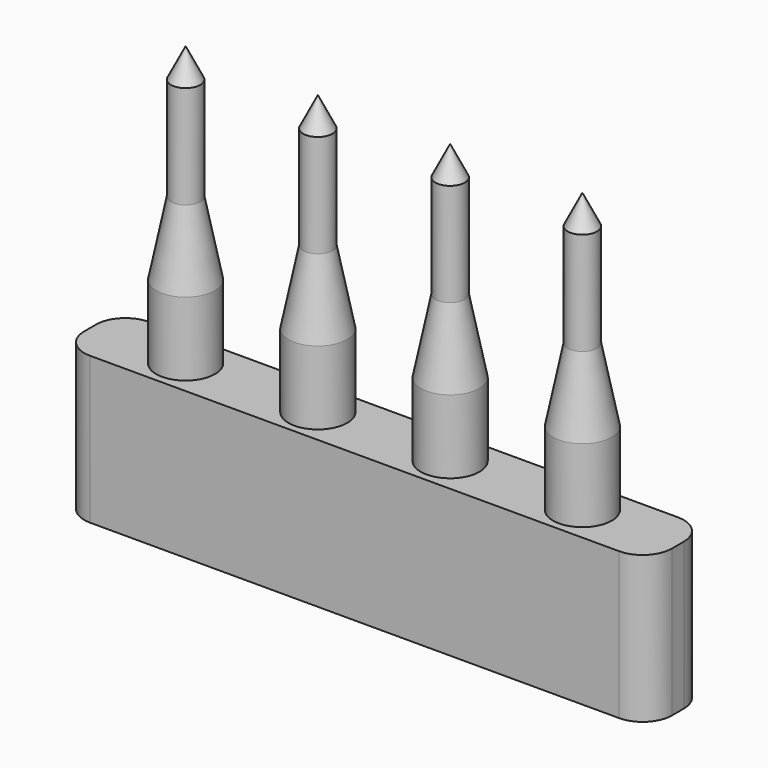
from build123d import *

# Parameters (mm, degrees)
F0_W     = 40
F0_H     = 5
F0_R     = 2
F0_R_2   = 1
F1_DEPTH = 10
F3_DEPTH = 5
F8_R     = 2


# Not quite as in the source:
# - a feature names something its author has since deleted; it is built from what else it names


with BuildPart() as f1:
    # F0 (on Top) → F1 (new body)
    with BuildSketch(Plane.XY):
        Rectangle(F0_W, F0_H)
        with Locations((-13.5, 0)):
            Circle(F0_R, mode=Mode.SUBTRACT)
        with BuildLine():
            ThreePointArc((-6.5, 0), (-4.5, 2), (-2.5, 0))
            ThreePointArc((-2.5, 0), (-4.5, -2), (-6.5, 0))
        make_face(mode=Mode.SUBTRACT)
        with BuildLine():
            ThreePointArc((6.5, 0), (4.5, -2), (2.5, 0))
            ThreePointArc((2.5, 0), (4.5, 2), (6.5, 0))
        make_face(mode=Mode.SUBTRACT)
        with BuildLine():
            ThreePointArc((15.5, 0), (13.5, -2), (11.5, 0))
            ThreePointArc((11.5, 0), (13.5, 2), (15.5, 0))
        make_face(mode=Mode.SUBTRACT)
        with BuildLine():
            ThreePointArc((15.5, 0), (13.5, 2), (11.5, 0))
            ThreePointArc((11.5, 0), (13.5, -2), (15.5, 0))
        make_face()
        with BuildLine():
            ThreePointArc((14.5, 0), (13.5, -1), (12.5, 0))
            ThreePointArc((12.5, 0), (13.5, 1), (14.5, 0))
        make_face(mode=Mode.SUBTRACT)
        with Locations((-13.5, 0)):
            Circle(F0_R)
        with Locations((-13.5, 0)):
            Circle(F0_R_2, mode=Mode.SUBTRACT)
        with BuildLine():
            ThreePointArc((14.5, 0), (13.5, 1), (12.5, 0))
            ThreePointArc((12.5, 0), (13.5, -1), (14.5, 0))
        make_face()
        with BuildLine():
            Line((4.5, 0), (3.5, 0))
            ThreePointArc((3.5, 0), (4.5, -1), (5.5, 0))
            Line((5.5, 0), (4.5, 0))
        make_face()
        with BuildLine():
            ThreePointArc((-5.5, 0), (-4.5, -1), (-3.5, 0))
            Line((-3.5, 0), (-4.5, 0))
            Line((-4.5, 0), (-5.5, 0))
        make_face()
        with Locations((-13.5, 0)):
            Circle(F0_R_2)
        with BuildLine():
            Line((-4.5, 0), (-3.5, 0))
            ThreePointArc((-3.5, 0), (-4.5, 1), (-5.5, 0))
            Line((-5.5, 0), (-4.5, 0))
        make_face()
        with BuildLine():
            ThreePointArc((5.5, 0), (4.5, 1), (3.5, 0))
            Line((3.5, 0), (4.5, 0))
            Line((4.5, 0), (5.5, 0))
        make_face()
        with BuildLine():
            ThreePointArc((-6.5, 0), (-4.5, -2), (-2.5, 0))
            Line((-2.5, 0), (-3.5, 0))
            ThreePointArc((-3.5, 0), (-4.5, -1), (-5.5, 0))
            Line((-5.5, 0), (-6.5, 0))
        make_face()
        with BuildLine():
            Line((3.5, 0), (2.5, 0))
            ThreePointArc((2.5, 0), (4.5, -2), (6.5, 0))
            Line((6.5, 0), (5.5, 0))
            ThreePointArc((5.5, 0), (4.5, -1), (3.5, 0))
        make_face()
        with BuildLine():
            ThreePointArc((6.5, 0), (4.5, 2), (2.5, 0))
            Line((2.5, 0), (3.5, 0))
            ThreePointArc((3.5, 0), (4.5, 1), (5.5, 0))
            Line((5.5, 0), (6.5, 0))
        make_face()
        with BuildLine():
            Line((-3.5, 0), (-2.5, 0))
            ThreePointArc((-2.5, 0), (-4.5, 2), (-6.5, 0))
            Line((-6.5, 0), (-5.5, 0))
            ThreePointArc((-5.5, 0), (-4.5, 1), (-3.5, 0))
        make_face()
    extrude(amount=-F1_DEPTH)

    # F0 (on Top) → F3 (join)
    with BuildSketch(Plane.XY):
        with Locations((-13.5, 0)):
            Circle(F0_R)
        with Locations((-13.5, 0)):
            Circle(F0_R_2, mode=Mode.SUBTRACT)
        with BuildLine():
            ThreePointArc((15.5, 0), (13.5, 2), (11.5, 0))
            ThreePointArc((11.5, 0), (13.5, -2), (15.5, 0))
        make_face()
        with BuildLine():
            ThreePointArc((14.5, 0), (13.5, -1), (12.5, 0))
            ThreePointArc((12.5, 0), (13.5, 1), (14.5, 0))
        make_face(mode=Mode.SUBTRACT)
        with BuildLine():
            Line((4.5, 0), (3.5, 0))
            ThreePointArc((3.5, 0), (4.5, -1), (5.5, 0))
            Line((5.5, 0), (4.5, 0))
        make_face()
        with BuildLine():
            ThreePointArc((14.5, 0), (13.5, 1), (12.5, 0))
            ThreePointArc((12.5, 0), (13.5, -1), (14.5, 0))
        make_face()
        with BuildLine():
            ThreePointArc((5.5, 0), (4.5, 1), (3.5, 0))
            Line((3.5, 0), (4.5, 0))
            Line((4.5, 0), (5.5, 0))
        make_face()
        with BuildLine():
            ThreePointArc((-5.5, 0), (-4.5, -1), (-3.5, 0))
            Line((-3.5, 0), (-4.5, 0))
            Line((-4.5, 0), (-5.5, 0))
        make_face()
        with BuildLine():
            Line((-4.5, 0), (-3.5, 0))
            ThreePointArc((-3.5, 0), (-4.5, 1), (-5.5, 0))
            Line((-5.5, 0), (-4.5, 0))
        make_face()
        with Locations((-13.5, 0)):
            Circle(F0_R_2)
        with BuildLine():
            ThreePointArc((-6.5, 0), (-4.5, -2), (-2.5, 0))
            Line((-2.5, 0), (-3.5, 0))
            ThreePointArc((-3.5, 0), (-4.5, -1), (-5.5, 0))
            Line((-5.5, 0), (-6.5, 0))
        make_face()
        with BuildLine():
            Line((-3.5, 0), (-2.5, 0))
            ThreePointArc((-2.5, 0), (-4.5, 2), (-6.5, 0))
            Line((-6.5, 0), (-5.5, 0))
            ThreePointArc((-5.5, 0), (-4.5, 1), (-3.5, 0))
        make_face()
        with BuildLine():
            ThreePointArc((6.5, 0), (4.5, 2), (2.5, 0))
            Line((2.5, 0), (3.5, 0))
            ThreePointArc((3.5, 0), (4.5, 1), (5.5, 0))
            Line((5.5, 0), (6.5, 0))
        make_face()
        with BuildLine():
            Line((3.5, 0), (2.5, 0))
            ThreePointArc((2.5, 0), (4.5, -2), (6.5, 0))
            Line((6.5, 0), (5.5, 0))
            ThreePointArc((5.5, 0), (4.5, -1), (3.5, 0))
        make_face()
    extrude(amount=F3_DEPTH)

    # F2 (on Front) → F4 (revolve)
    with BuildSketch(Plane.XZ):
        Polygon((-13.5, 19), (-13.5, 10), (-12.5, 10), (-12.5, 17), align=None)
        Polygon((-13.5, 10), (-13.5, 5), (-11.5, 5), (-12.5, 10), align=None)
    revolve(axis=Axis((-13.5, 0, 14.5), (0, 0, 1)))

    # F2 (on Front) → F5 (revolve)
    with BuildSketch(Plane.XZ):
        Polygon((-4.5, 19), (-4.5, 10), (-3.5, 10), (-3.5, 17), align=None)
        Polygon((-4.5, 10), (-4.5, 5), (-2.5, 5), (-3.5, 10), align=None)
    revolve(axis=Axis((-4.5, 0, 14.5), (0, 0, 1)))

    # F2 (on Front) → F6 (revolve)
    with BuildSketch(Plane.XZ):
        Polygon((2.5, 5), (4.5, 5), (4.5, 10), (3.5, 10), align=None)
        Polygon((3.5, 10), (4.5, 10), (4.5, 19), (3.5, 17), align=None)
    revolve(axis=Axis((4.5, 0, 14.5), (0, 0, 1)))

    # F2 (on Front) → F7 (revolve)
    with BuildSketch(Plane.XZ):
        Polygon((13.5, 5), (13.5, 10), (13.5, 19), (12.5, 17), (12.5, 10), (11.5, 5), align=None)
    revolve(axis=Axis((13.5, 0, 14.5), (0, 0, 1)))

    # F8
    f8_edges = [f1.edges().sort_by_distance(p)[0] for p in [
        (-20, -2.5, -5),
        (-20, 2.5, -5),
        (20, -2.5, -5),
        (20, 2.5, -5),
    ]]
    fillet(f8_edges, radius=F8_R)


solid = f1.part
